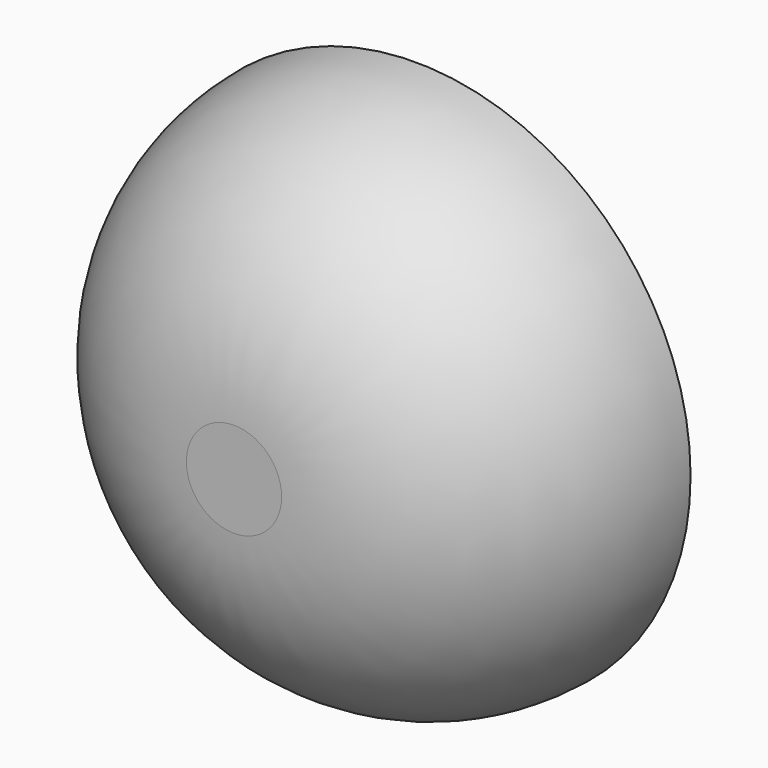
from build123d import *

# Parameters (mm, degrees)
F0_R     = 30.7226315835
F1_DEPTH = 25.4
F2_R     = 25.39999


# Not quite as in the source:
# - a fillet or chamfer is up to 0.001 mm smaller than in the source, because OpenCascade refuses the exact size


with BuildPart() as f1:
    # F0 (on Front) → F1 (new body)
    with BuildSketch(Plane.XZ):
        Circle(F0_R)
    extrude(amount=F1_DEPTH)

    # F2 (radius 25.4 in the source; OpenCascade refuses exactly that, so slightly less here)
    f2_edges = [f1.edges().sort_by_distance(p)[0] for p in [
        (-30.722632, -25.4, 0),
    ]]
    fillet(f2_edges, radius=F2_R)


solid = f1.part
